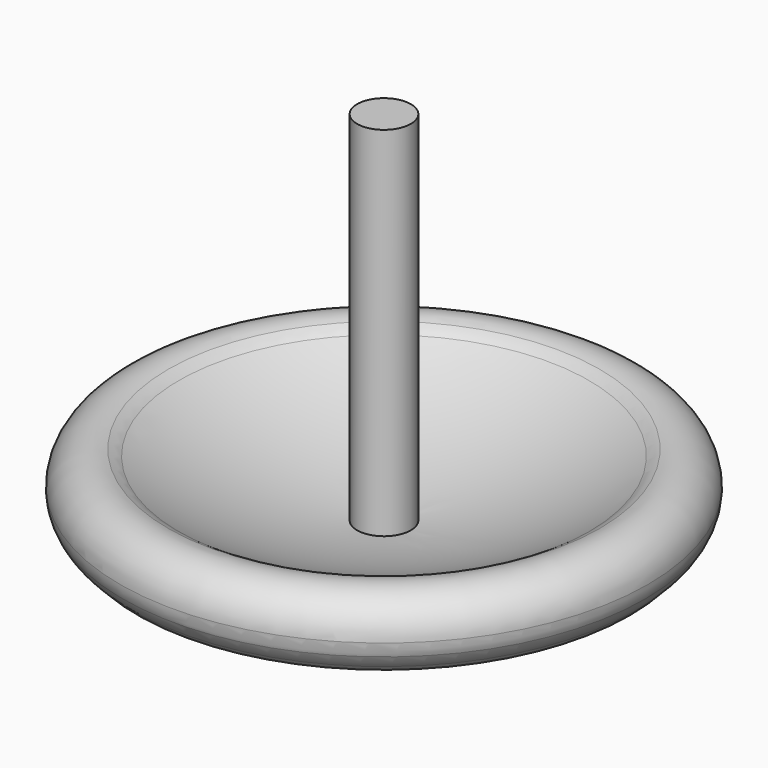
from build123d import *


# Not quite as in the source:
# - a fillet or chamfer that OpenCascade refuses, or shapes differently, is made with other operations: its cross-section is extruded or revolved along the edge and cut away or added


with BuildPart() as f1:
    # F0 (on Front) → F1 (revolve)
    with BuildSketch(Plane.XZ):
        with BuildLine():
            ThreePointArc((72.7515336349, 31.5465186996), (42.1923391821, 18.1752933834), (9.525, 11.43))
            Line((9.525, 11.43), (9.525, 138.43))
            Line((9.525, 138.43), (0, 138.43))
            Line((0, 138.43), (0, 5.08))
            Line((0, 5.08), (8.89, 5.08))
            Line((8.89, 5.08), (80.9900359946, 5.08))
            ThreePointArc((80.9900359946, 5.08), (85.3313804759, 8.3219837991), (89.1588856559, 12.1570763605))
            ThreePointArc((89.1588856559, 12.1570763605), (71.2952522719, 13.6775386544), (72.7515336349, 31.5465186996))
        make_face()
        with BuildLine():
            ThreePointArc((76.5693657258, 33.7870508297), (74.5620768343, 32.8344105725), (72.7515336349, 31.5465186996))
            ThreePointArc((72.7515336349, 31.5465186996), (74.6681976781, 32.6535822964), (76.5693657258, 33.7870508297))
        make_face()
        with BuildLine():
            ThreePointArc((76.5693657258, 33.7870508297), (74.6681976781, 32.6535822964), (72.7515336349, 31.5465186996))
            ThreePointArc((72.7515336349, 31.5465186996), (71.2952522719, 13.6775386544), (89.1588856559, 12.1570763605))
            ThreePointArc((89.1588856559, 12.1570763605), (91.0491403746, 14.536624633), (92.7400229866, 17.0617442093))
            ThreePointArc((92.7400229866, 17.0617442093), (93.4502694354, 19.4251359639), (93.6900359946, 21.8812675974))
            ThreePointArc((93.6900359946, 21.8812675974), (88.2408113871, 32.3079763881), (76.5693657258, 33.7870508297))
        make_face()
        with BuildLine():
            ThreePointArc((92.7400229866, 17.0617442093), (91.0491403746, 14.536624633), (89.1588856559, 12.1570763605))
            ThreePointArc((89.1588856559, 12.1570763605), (91.2469339214, 14.3922059126), (92.7400229866, 17.0617442093))
        make_face()
        Polygon((8.89, 5.08), (0, 5.08), (0, 0), (0, -6.35), align=None)
    revolve(axis=Axis((0, 0, 4.7224786045), (0, 0, 1)))

    # F2: chamfer of 5.08 on 1 edges, made by hand

    # F2_s1 → F2_t2 (revolve, cut)
    with BuildSketch(Plane.XZ):
        with BuildLine():
            Line((74.8406610891, 5.0020764693), (87.521834843, 10.2676383795))
            Line((87.521834843, 10.2676383795), (87.5938009931, 10.1959206464))
            ThreePointArc((87.5938009931, 10.1959206464), (84.4417917383, 7.4442968535), (81.044772889, 4.9944054185))
            Line((81.044772889, 4.9944054185), (80.9900359946, 4.9784))
            ThreePointArc((80.9900359946, 4.9784), (77.9153485418, 4.9784), (74.8406610891, 4.9004764693))
            Line((74.8406610891, 4.9004764693), (74.8406610891, 5.0020764693))
        make_face()
    revolve(axis=Axis((0, 0, 5.08), (0, 0, 1)), mode=Mode.SUBTRACT)


solid = f1.part
